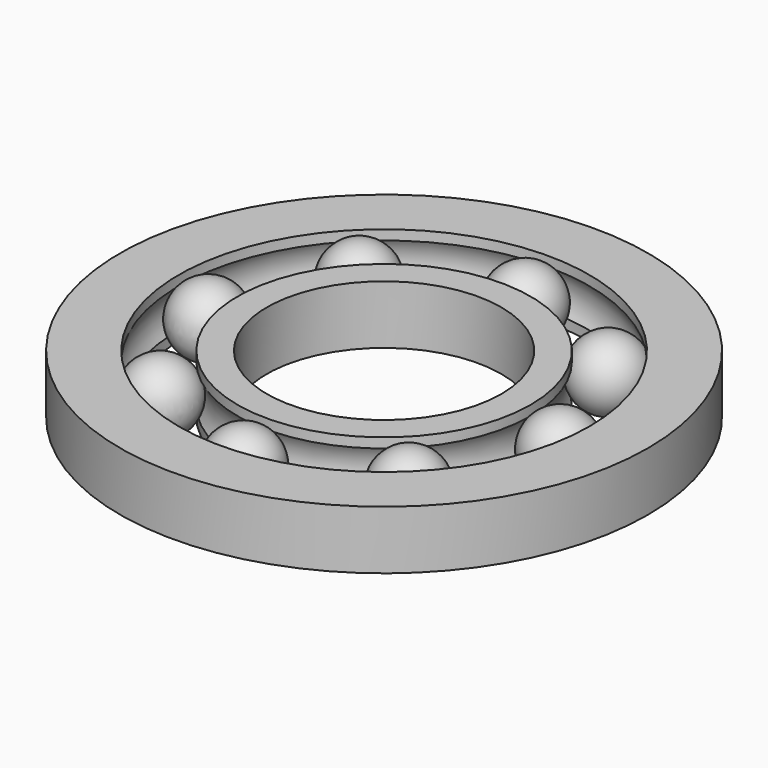
from build123d import *

# Parameters (mm, degrees)
F0_R     = 45
F0_R_2   = 35
F3_DEPTH = 5
F0_R_3   = 25
F0_R_4   = 20
F6_COUNT = 8


with BuildPart() as f2:
    # F1 (on Top) → F2 (revolve)
    with BuildSketch(Plane.XY):
        with BuildLine():
            ThreePointArc((0, 36), (-6, 30), (0, 24))
            Line((0, 24), (0, 36))
        make_face()
    revolve(axis=Axis((0, 30, 0), (0, 1, 0)))


with BuildPart() as f3:
    # F0 (on Top) → F3 (new body, symmetric)
    with BuildSketch(Plane.XY):
        Circle(F0_R)
        Circle(F0_R_2, mode=Mode.SUBTRACT)
    extrude(amount=F3_DEPTH, both=True)


with BuildPart() as f3b:
    # F0 (on Top) → F3, piece 2 (new body, symmetric)
    with BuildSketch(Plane.XY):
        Circle(F0_R_3)
        Circle(F0_R_4, mode=Mode.SUBTRACT)
    extrude(amount=F3_DEPTH, both=True)


with BuildPart() as f5_tool:
    # F4 (on Right) → F5 (revolve)
    with BuildSketch(Plane.YZ):
        with BuildLine():
            Line((25, -3.3166247904), (25, 3.3166247904))
            ThreePointArc((25, 3.3166247904), (24, 0), (25, -3.3166247904))
        make_face()
        with BuildLine():
            ThreePointArc((35, -3.3166247904), (36, 0), (35, 3.3166247904))
            Line((35, 3.3166247904), (35, -3.3166247904))
        make_face()
    revolve(axis=Axis((0, 0, 5), (0, 0, 1)))


with BuildPart() as f3_1:
    add(f3.part)

    # F5: cut by f5_tool
    add(f5_tool.part, mode=Mode.SUBTRACT)


with BuildPart() as f3b_1:
    add(f3b.part)

    # F5: cut by f5_tool
    add(f5_tool.part, mode=Mode.SUBTRACT)


with BuildPart() as f6_1:
    # F6: instance of F2
    add(f2.part.rotate(Axis((0, 0, 5), (0, 0, 1)), 1 * 360 / F6_COUNT))


with BuildPart() as f6_2:
    # F6: instance of F2
    add(f2.part.rotate(Axis((0, 0, 5), (0, 0, 1)), 2 * 360 / F6_COUNT))


with BuildPart() as f6_3:
    # F6: instance of F2
    add(f2.part.rotate(Axis((0, 0, 5), (0, 0, 1)), 3 * 360 / F6_COUNT))


with BuildPart() as f6_4:
    # F6: instance of F2
    add(f2.part.rotate(Axis((0, 0, 5), (0, 0, 1)), 4 * 360 / F6_COUNT))


with BuildPart() as f6_5:
    # F6: instance of F2
    add(f2.part.rotate(Axis((0, 0, 5), (0, 0, 1)), 5 * 360 / F6_COUNT))


with BuildPart() as f6_6:
    # F6: instance of F2
    add(f2.part.rotate(Axis((0, 0, 5), (0, 0, 1)), 6 * 360 / F6_COUNT))


with BuildPart() as f6_7:
    # F6: instance of F2
    add(f2.part.rotate(Axis((0, 0, 5), (0, 0, 1)), 7 * 360 / F6_COUNT))


solid = Compound([f2.part, f3_1.part, f3b_1.part, f6_1.part, f6_2.part, f6_3.part, f6_4.part, f6_5.part, f6_6.part, f6_7.part])
